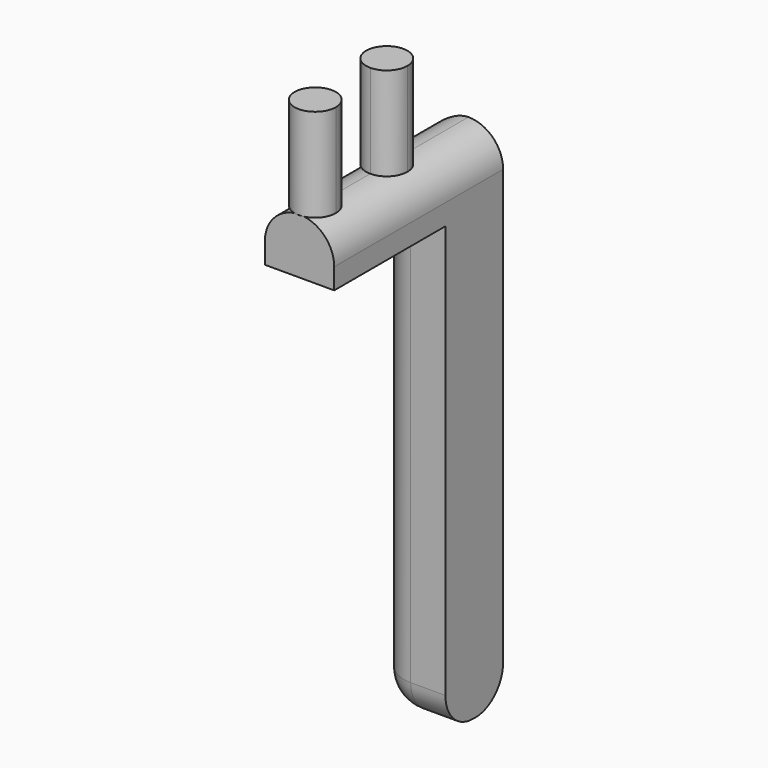
from build123d import *

# Parameters (mm, degrees)
F1_DEPTH      = 6.8326
F2_W          = 15.4686
F2_H          = 4.064
F3_DEPTH      = 2.54
F3_DEPTH_BACK = 2.54
F4_W          = 5.2863146343
F4_H          = 32.8
F5_DEPTH      = 2.54
F5_DEPTH_BACK = 2.54
F6_R          = 2.54
F7_R          = 2.53999


# Not quite as in the source:
# - a fillet or chamfer is up to 0.001 mm smaller than in the source, because OpenCascade refuses the exact size


with BuildPart() as f1:
    # F0 (on Top) → F1 (new body)
    with BuildSketch(Plane.XY):
        with BuildLine():
            ThreePointArc((0, 5.0419), (1.0686504784, 5.4845495216), (1.5113, 6.5532))
            ThreePointArc((1.5113, 6.5532), (-1.0686504784, 7.6218504784), (0, 5.0419))
        make_face()
    extrude(amount=F1_DEPTH)


with BuildPart() as f1b:
    # F0 (on Top) → F1, piece 2 (new body)
    with BuildSketch(Plane.XY):
        with BuildLine():
            ThreePointArc((1.5113, 0), (1.0686504784, 1.0686504784), (0, 1.5113))
            ThreePointArc((0, 1.5113), (-1.0686504784, -1.0686504784), (1.5113, 0))
        make_face()
    extrude(amount=F1_DEPTH)


with BuildPart() as f3:
    # F2 (on Right) → F3 (new body, two sides)
    with BuildSketch(Plane.YZ) as f3_sk:
        with Locations((6.2986569509, -2.032)):
            Rectangle(F2_W, F2_H)
    extrude(amount=F3_DEPTH)
    extrude(f3_sk.sketch, amount=-F3_DEPTH_BACK)

    # F4 (on Right) → F5 (join, two sides)
    with BuildSketch(Plane.YZ) as f5_sk:
        with Locations((11.3897996337, -20.464)):
            Rectangle(F4_W, F4_H)
    extrude(amount=F5_DEPTH)
    extrude(f5_sk.sketch, amount=-F5_DEPTH_BACK)

    # F6
    f6_edges = [f3.edges().sort_by_distance(p)[0] for p in [
        (0, 8.746642, -36.864),
        (0, 14.032957, -36.864),
    ]]
    fillet(f6_edges, radius=F6_R)

    # F7 (radius 2.54 in the source; OpenCascade refuses exactly that, so slightly less here)
    f7_edges = [f3.edges().sort_by_distance(p)[0] for p in [
        (2.54, 6.298657, 0),
        (-2.54, 6.298657, 0),
        (-2.54, 14.032957, -17.162),
    ]]
    fillet(f7_edges, radius=F7_R)


solid = Compound([f1.part, f1b.part, f3.part])
